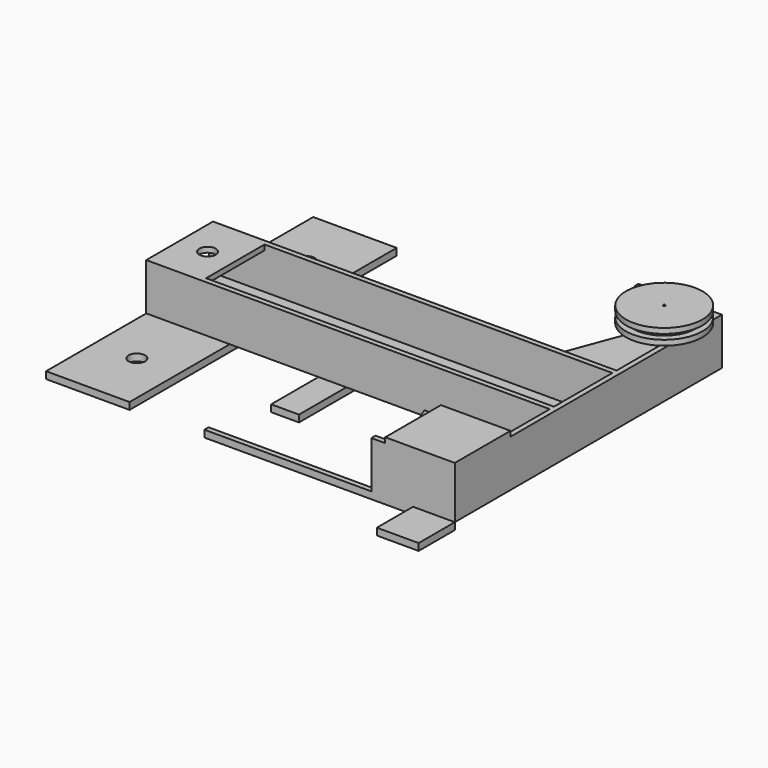
from build123d import *

# Parameters (mm, degrees)
F0_W      = 476.4060080051
F0_H      = 19.05
F0_H_2    = 266.7
F0_W_2    = 1016
F0_R      = 30.1244
F1_DEPTH  = 19.05
F2_W      = 19.05
F2_H      = 1219.2
F3_DEPTH  = 152.4
F4_W      = 285.75
F4_H      = 19.05
F5_DEPTH  = 152.4
F7_DEPTH  = 152.4
F8_W      = 203.2
F8_H      = 266.7
F8_R      = 30.1244
F9_DEPTH  = 19.05
F11_DEPTH = 19.05
F12_R     = 139.7
F13_DEPTH = 19.05
F14_R     = 114.3
F15_DEPTH = 19.05
F16_R     = 139.7
F17_DEPTH = 19.05
F18_W     = 101.6
F18_H     = 736.6
F20_DEPTH = 25.4
F21_R     = 3.9878
F22_DEPTH = 96.52
F23_W     = 304.8
F23_H     = 457.2
F23_R     = 30.1244
F23_H_2   = 304.8
F24_DEPTH = 25.4
F25_W     = 254
F25_H     = 254
F26_DEPTH = 19.05
F28_DEPTH = 25.4
F29_W     = 152.4
F29_H     = 25.4
F30_DEPTH = 165.1


# Not quite as in the source:
# - a feature of the source that left no trace in its solid (it failed there, or was rolled back) is left out


with BuildPart() as f1:
    # F0 (on Top) → F1 (new body)
    with BuildSketch(Plane.XY):
        Polygon((-304.8, 0), (0, 0), (0, 457.2), (-476.4060080051, 457.2), align=None)
        with Locations((-238.2030040026, 466.725)):
            Rectangle(F0_W, F0_H)
        with Locations((-238.2030040026, 609.6)):
            Rectangle(F0_W, F0_H_2)
        with Locations((-984.4060080051, 466.725)):
            Rectangle(F0_W_2, F0_H)
        Polygon((-476.4060080051, 742.95), (0, 742.95), (0, 762), (0, 1219.2), (-304.8, 1219.2), (-476.4060080051, 762), align=None)
        with Locations((-984.4060080051, 609.6)):
            Rectangle(F0_W_2, F0_H_2)
        with Locations((-1389.0752792358, 609.6)):
            Circle(F0_R, mode=Mode.SUBTRACT)
        with Locations((-984.4060080051, 752.475)):
            Rectangle(F0_W_2, F0_H)
    extrude(amount=F1_DEPTH)

    # F2 (on face) → F3 (join)
    with BuildSketch(Plane.XY.offset(19.05)):
        with Locations((-9.525, 609.6)):
            Rectangle(F2_W, F2_H)
    extrude(amount=F3_DEPTH)

    # F4 (on face) → F5 (join)
    with BuildSketch(Plane.XY.offset(19.05)):
        with Locations((-161.925, 9.525)):
            Rectangle(F4_W, F4_H)
        with Locations((-161.925, 1209.675)):
            Rectangle(F4_W, F4_H)
    extrude(amount=F5_DEPTH)

    # F6 (on face) → F7 (join)
    with BuildSketch(Plane.XY.offset(19.05)):
        Polygon((-476.4060080051, 762), (-1492.4060080051, 762), (-1492.4060080051, 742.95), (-19.05, 742.95), (-19.05, 762), align=None)
        Polygon((-19.05, 476.25), (-1492.4060080051, 476.25), (-1492.4060080051, 457.2), (-476.4060080051, 457.2), (-19.05, 457.2), align=None)
    extrude(amount=F7_DEPTH)

    # F8 (on face) → F9 (join)
    with BuildSketch(Plane.XY.offset(171.45)):
        with Locations((-1390.8060080051, 609.6)):
            Rectangle(F8_W, F8_H)
        with Locations((-1388.1880044937, 606.7718267441)):
            Circle(F8_R, mode=Mode.SUBTRACT)
        Polygon((-1492.4060080051, 762), (-1492.4060080051, 742.95), (-1289.2060080051, 742.95), (-19.05, 742.95), (-19.05, 476.25), (-1289.2060080051, 476.25), (-1492.4060080051, 476.25), (-1492.4060080051, 457.2), (-19.05, 457.2), (-19.05, 19.05), (-304.8, 19.05), (-304.8, 0), (0, 0), (0, 1219.2), (-304.8, 1219.2), (-304.8, 1200.15), (-19.05, 1200.15), (-19.05, 762), align=None)
    extrude(amount=-F9_DEPTH)

    # F12 (on face) → F13 (join)
    with BuildSketch(Plane.XY.offset(171.45)):
        with Locations((-95.896191895, 1075.6877660751)):
            Circle(F12_R)
    extrude(amount=F13_DEPTH)

    # F14 (on face) → F15 (join)
    with BuildSketch(Plane.XY.offset(190.5)):
        with Locations((-95.896191895, 1075.6877660751)):
            Circle(F14_R)
    extrude(amount=F15_DEPTH)

    # F16 (on face) → F17 (join)
    with BuildSketch(Plane.XY.offset(209.55)):
        with Locations((-95.896191895, 1075.6877660751)):
            Circle(F16_R)
    extrude(amount=F17_DEPTH)

    # F18 (on face) → F20 (join)
    with BuildSketch(Plane(origin=(0, 0, 0), x_dir=(1, 0, 0), z_dir=(0, 0, -1))):
        with Locations((-812.8, -609.6)):
            Rectangle(F18_W, F18_H)
    extrude(amount=F20_DEPTH)


with BuildPart() as f11:
    # F10 (on face) → F11 (new body)
    with BuildSketch(Plane.XY.offset(171.45)):
        Polygon((-19.05, 981.71), (-19.05, 1019.81), (-199.39, 1200.15), (-237.49, 1200.15), align=None)
    extrude(amount=-F11_DEPTH)


with BuildPart() as f22_tool:
    # F21 (on face) → F22 (new body)
    with BuildSketch(Plane.XY.offset(228.6)):
        with Locations((-95.896191895, 1075.6877660751)):
            Circle(F21_R)
    extrude(amount=-F22_DEPTH)


with BuildPart() as f1_1:
    add(f1.part)

    # F22: cut by f22_tool
    add(f22_tool.part, mode=Mode.SUBTRACT)

    # F23 (on face) → F24 (join)
    with BuildSketch(Plane(origin=(0, 0, 0), x_dir=(1, 0, 0), z_dir=(0, 0, -1))):
        with Locations((-1340.0060080051, -990.6)):
            Rectangle(F23_W, F23_H)
        with Locations((-1338.4050130844, -995.3244)):
            Circle(F23_R, mode=Mode.SUBTRACT)
        with Locations((-1340.0060080051, -609.6)):
            Rectangle(F23_W, F23_H_2)
        with Locations((-1389.0752792358, -609.6)):
            Circle(F23_R, mode=Mode.SUBTRACT)
        with Locations((-1340.0060080051, -228.6)):
            Rectangle(F23_W, F23_H)
        with Locations((-1340.0060080051, -223.8756)):
            Circle(F23_R, mode=Mode.SUBTRACT)
    extrude(amount=F24_DEPTH)

    # F25 (on face) → F26 (join)
    with BuildSketch(Plane.XY.offset(171.45)):
        with Locations((-127, 127)):
            Rectangle(F25_W, F25_H)
    extrude(amount=F26_DEPTH)

    # F27 (on face) → F28 (join)
    with BuildSketch(Plane(origin=(0, 0, 0), x_dir=(1, 0, 0), z_dir=(0, 0, -1))):
        Polygon((-152.4, 0), (-304.8, 0), (-914.4, 0), (-914.4, -19.05), (-152.4, -19.05), align=None)
    extrude(amount=F28_DEPTH)


with BuildPart() as f11_1:
    add(f11.part)

    # F22: cut by f22_tool
    add(f22_tool.part, mode=Mode.SUBTRACT)


with BuildPart() as f30:
    # F29 (on face) → F30 (new body)
    with BuildSketch(Plane.XZ):
        with Locations((-76.2, -12.7)):
            Rectangle(F29_W, F29_H)
    extrude(amount=F30_DEPTH)


solid = Compound([f1_1.part, f11_1.part, f30.part])
